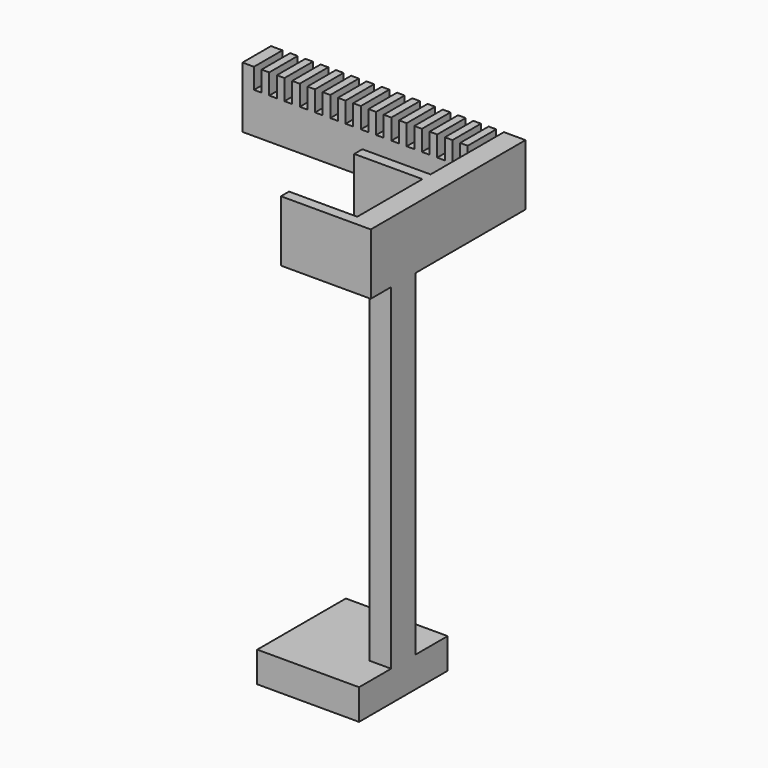
from build123d import *

# Parameters (mm, degrees)
F0_W     = 2.8575
F0_H     = 5.08
F0_W_2   = 1.905
F0_W_3   = 5.3975
F0_H_2   = 5.128411484
F1_DEPTH = 4.445
F2_W     = 7.62
F2_H     = 83.82
F3_DEPTH = 5.3975
F4_W     = 17.018
F4_H     = 2.54
F4_W_2   = 2.45618
F4_W_3   = 14.56182
F5_DEPTH = 15.24
F6_DEPTH = 25.4


# Not quite as in the source:
# - a feature names something its author has since deleted; it is built from what else it names


with BuildPart() as f1:
    # F0 (on Front) → F1 (new body, symmetric)
    with BuildSketch(Plane.XZ):
        with Locations((-63.4578398415, 18.0266693214)):
            Rectangle(F0_W, F0_H)
        Polygon((-62.0290898415, 15.4866693214), (-64.8865898415, 15.4866693214), (-64.8865898415, 5.3266693214), (-1.3865898415, 5.3266693214), (-1.3865898415, 15.4866693214), (-6.7840898415, 15.4866693214), (-8.6890898415, 15.4866693214), (-10.5940898415, 15.4866693214), (-12.4990898415, 15.4866693214), (-13.314443469, 15.4866693214), (-14.4040898415, 15.4866693214), (-16.3090898415, 15.4866693214), (-18.2140898415, 15.4866693214), (-20.1190898415, 15.4866693214), (-22.0240898415, 15.4866693214), (-23.9290898415, 15.4866693214), (-25.8340898415, 15.4866693214), (-27.7390898415, 15.4866693214), (-29.6440898415, 15.4866693214), (-31.5490898415, 15.4866693214), (-33.4540898415, 15.4866693214), (-35.3590898415, 15.4866693214), (-37.2640898415, 15.4866693214), (-39.1690898415, 15.4866693214), (-41.0740898415, 15.4866693214), (-42.9790898415, 15.4866693214), (-44.8840898415, 15.4866693214), (-46.7890898415, 15.4866693214), (-48.6940898415, 15.4866693214), (-50.5990898415, 15.4866693214), (-52.5040898415, 15.4866693214), (-54.4090898415, 15.4866693214), (-56.3140898415, 15.4866693214), (-58.2190898415, 15.4866693214), (-60.1240898415, 15.4866693214), align=None)
        with Locations((-59.1715898415, 18.0266693214)):
            Rectangle(F0_W_2, F0_H)
        with Locations((-4.0853398415, 18.0266693214)):
            Rectangle(F0_W_3, F0_H)
        with Locations((-55.3615898415, 18.0266693214)):
            Rectangle(F0_W_2, F0_H)
        with Locations((-9.6415898415, 18.0266693214)):
            Rectangle(F0_W_2, F0_H)
        with Locations((-51.5515898415, 18.0266693214)):
            Rectangle(F0_W_2, F0_H)
        Polygon((-13.314443469, 15.4866693214), (-12.4990898415, 15.4866693214), (-12.4990898415, 20.5666693214), (-13.314443469, 20.5666693214), (-14.4040898415, 20.5666693214), (-14.4040898415, 15.4866693214), align=None)
        with Locations((-47.7415898415, 18.0266693214)):
            Rectangle(F0_W_2, F0_H)
        with Locations((-43.9315898415, 18.0266693214)):
            Rectangle(F0_W_2, F0_H)
        with Locations((-17.2615898415, 18.0266693214)):
            Rectangle(F0_W_2, F0_H)
        with Locations((-40.1215898415, 18.0266693214)):
            Rectangle(F0_W_2, F0_H)
        with Locations((-21.0715898415, 18.0266693214)):
            Rectangle(F0_W_2, F0_H)
        with Locations((-36.3115898415, 18.0508750634)):
            Rectangle(F0_W_2, F0_H_2)
        with Locations((-24.8815898415, 18.0266693214)):
            Rectangle(F0_W_2, F0_H)
        with Locations((-32.5015898415, 18.0266693214)):
            Rectangle(F0_W_2, F0_H)
        with Locations((-28.6915898415, 18.0266693214)):
            Rectangle(F0_W_2, F0_H)
    extrude(amount=F1_DEPTH, both=True)

    # F2 (on face) → F3 (join)
    with BuildSketch(Plane.YZ.offset(-1.3865898415)):
        Polygon((-4.445, 5.3266693214), (-4.445, 20.5666693214), (-43.815, 20.5666693214), (-43.815, 5.3266693214), (-37.465, 5.3266693214), (-29.845, 5.3266693214), align=None)
        with Locations((-33.655, -36.5833306786)):
            Rectangle(F2_W, F2_H)
    extrude(amount=-F3_DEPTH)

    # F4 (on face) → F5 (join)
    with BuildSketch(Plane.XY.offset(20.5666693214)):
        with Locations((-15.2930898415, -19.685)):
            Rectangle(F4_W, F4_H)
        with Locations((-22.5739998415, -42.545)):
            Rectangle(F4_W_2, F4_H)
        with Locations((-14.0649998415, -42.545)):
            Rectangle(F4_W_3, F4_H)
    extrude(amount=-F5_DEPTH)

    # F2 (on face) → F6 (join)
    with BuildSketch(Plane.YZ.offset(-1.3865898415)):
        Polygon((-19.840323447, -78.4933306786), (-29.845, -78.4933306786), (-37.465, -78.4933306786), (-47.469676553, -78.4933306786), (-47.469676553, -86.1133306786), (-19.840323447, -86.1133306786), align=None)
    extrude(amount=-F6_DEPTH)


solid = f1.part
